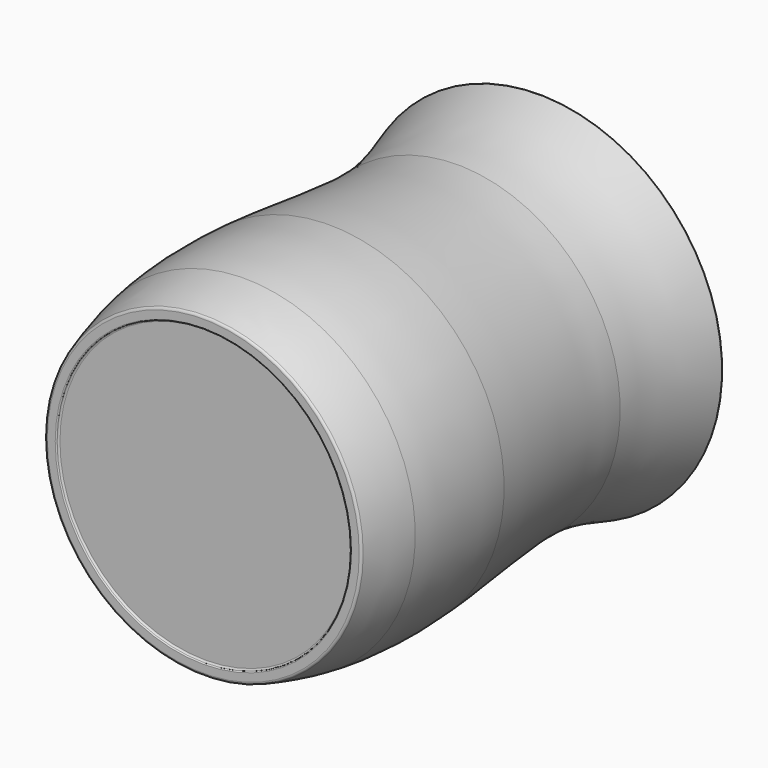
from build123d import *


with BuildPart() as f1:
    # F0 (on Top) → F1 (revolve)
    with BuildSketch(Plane.XY):
        with BuildLine():
            Line((-14.6370422903, 10.1036671021), (13.0629577097, 10.1036671021))
            Line((13.0629577097, 10.1036671021), (13.0629577097, 12.6036671021))
            Line((13.0629577097, 12.6036671021), (-14.1784562304, 12.6038035398))
            ThreePointArc((-14.1784562304, 12.6038035398), (-16.2147681614, 13.4007664255), (-17.1691759328, 15.3682068762))
            add(Edge.make_bspline(
                [(-20.883924226, 89.4849003641), (-18.2263420174, 83.5118232537), (-12.3246366266, 70.1591899551), (-18.201164969, 40.4058481236), (-17.6432060424, 21.9639149031), (-17.2642566255, 16.5751897143), (-17.1691759328, 15.3682068762)],
                knots=[0.0017323014, 0.0017323014, 0.0017323014, 0.0017323014, 0.263245612, 0.5854099201, 0.8471807154, 0.9319391838, 0.9319391838, 0.9319391838, 0.9319391838], degree=3))
            ThreePointArc((-20.883924226, 89.4849003641), (-20.9577048707, 89.5713194622), (-21.0666538075, 89.6035990723))
            Line((-21.0666538075, 89.6035990723), (-21.6655251791, 89.6035990723))
            ThreePointArc((-21.6655251791, 89.6035990723), (-21.8264908594, 89.5223005877), (-21.8565938809, 89.3444995699))
            add(Edge.make_bspline(
                [(-17.9370422782, 70.1036666905), (-18.1926220786, 77.4573838205), (-20.0205935681, 83.4087102326), (-21.8565938809, 89.3444995699)],
                knots=[0.7468257278, 0.7468257278, 0.7468257278, 0.7468257278, 0.9963690343, 0.9963690343, 0.9963690343, 0.9963690343], degree=3))
            add(Edge.make_bspline(
                [(-20.2370421016, 39.6036670984), (-19.6019652652, 49.4001033217), (-17.5753267132, 60.8564073711), (-17.9370422798, 70.1036667357)],
                knots=[0.4344350208, 0.4344350208, 0.4344350208, 0.4344350208, 0.7474683162, 0.7474683162, 0.7474683162, 0.7474683162], degree=3))
            add(Edge.make_bspline(
                [(-19.4441677957, 19.4406417091), (-19.849904935, 24.8158820913), (-20.6073778309, 31.6554394078), (-20.2370421046, 39.6036670568)],
                knots=[0.1780933018, 0.1780933018, 0.1780933018, 0.1780933018, 0.4329958924, 0.4329958924, 0.4329958924, 0.4329958924], degree=3))
            add(Edge.make_bspline(
                [(-17.1166194806, 9.9618388722), (-17.9764397241, 12.8685379122), (-18.8271293588, 15.8029613087), (-19.4441677932, 19.4406416767)],
                knots=[0.0071105369, 0.0071105369, 0.0071105369, 0.0071105369, 0.1801794053, 0.1801794053, 0.1801794053, 0.1801794053], degree=3))
            ThreePointArc((-17.1166194806, 9.9618388722), (-16.9363937644, 9.7030961877), (-16.6371564964, 9.6036671021))
            Line((-16.6371564964, 9.6036671021), (-15.1370422903, 9.6036671021))
            ThreePointArc((-15.1370422903, 9.6036671021), (-14.9956209341, 9.6622457458), (-14.9370422903, 9.8036671021))
            ThreePointArc((-14.9370422903, 9.8036671021), (-14.8491743247, 10.0157991364), (-14.6370422903, 10.1036671021))
        make_face()
        with BuildLine():
            add(Edge.make_bspline(
                [(-19.4441677932, 19.4406416767), (-20.3506594604, 24.7847608711), (-20.7528717412, 31.6466894915), (-20.2370421016, 39.6036670984)],
                knots=[0.1801794053, 0.1801794053, 0.1801794053, 0.1801794053, 0.4344350208, 0.4344350208, 0.4344350208, 0.4344350208], degree=3))
            add(Edge.make_bspline(
                [(-19.4441677957, 19.4406417091), (-19.849904935, 24.8158820913), (-20.6073778309, 31.6554394078), (-20.2370421046, 39.6036670568)],
                knots=[0.1780933018, 0.1780933018, 0.1780933018, 0.1780933018, 0.4329958924, 0.4329958924, 0.4329958924, 0.4329958924], degree=3))
        make_face()
    revolve(axis=Axis((13.0629577097, 9.8536671021, 0), (0, 1, 0)))


solid = f1.part
